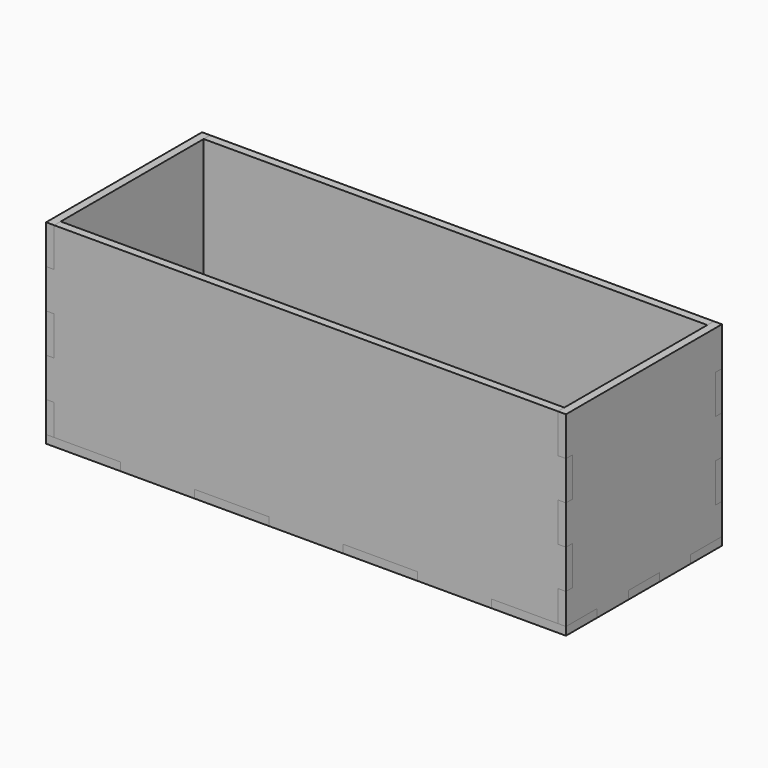
from build123d import *

# Parameters (mm, degrees)
F0_W     = 3.175
F0_H     = 3.175
F0_H_2   = 12.065
F0_W_2   = 25.8535714286
F0_H_3   = 15.24
F0_W_3   = 29.0285714286
F1_DEPTH = 3.175
F2_W     = 3.175
F2_H     = 15.24
F2_H_2   = 12.065
F2_H_3   = 3.175
F3_DEPTH = 3.175
F7_DEPTH = 3.175


with BuildPart() as f1:
    # F0 (on Top) → F1 (new body)
    with BuildSketch(Plane.XY):
        with Locations((-100.0125, 36.5125)):
            Rectangle(F0_W, F0_H)
        with Locations((-100.0125, 28.8925)):
            Rectangle(F0_W, F0_H_2)
        with Locations((-85.4982142857, 36.5125)):
            Rectangle(F0_W_2, F0_H)
        Polygon((98.425, 22.86), (98.425, 34.925), (72.5714285714, 34.925), (43.5428571429, 34.925), (14.5142857143, 34.925), (-14.5142857143, 34.925), (-43.5428571429, 34.925), (-72.5714285714, 34.925), (-98.425, 34.925), (-98.425, 22.86), (-98.425, 7.62), (-98.425, -7.62), (-98.425, -22.86), (-98.425, -34.925), (-72.5714285714, -34.925), (-43.5428571429, -34.925), (-14.5142857143, -34.925), (14.5142857143, -34.925), (43.5428571429, -34.925), (72.5714285714, -34.925), (98.425, -34.925), (98.425, -22.86), (98.425, -7.62), (98.425, 7.62), align=None)
        with Locations((-100.0125, 0)):
            Rectangle(F0_W, F0_H_3)
        with Locations((-100.0125, -28.8925)):
            Rectangle(F0_W, F0_H_2)
        with Locations((-100.0125, -36.5125)):
            Rectangle(F0_W, F0_H)
        with Locations((-85.4982142857, -36.5125)):
            Rectangle(F0_W_2, F0_H)
        with Locations((-29.0285714286, -36.5125)):
            Rectangle(F0_W_3, F0_H)
        with Locations((29.0285714286, -36.5125)):
            Rectangle(F0_W_3, F0_H)
        with Locations((85.4982142857, -36.5125)):
            Rectangle(F0_W_2, F0_H)
        with Locations((100.0125, -36.5125)):
            Rectangle(F0_W, F0_H)
        with Locations((100.0125, -28.8925)):
            Rectangle(F0_W, F0_H_2)
        with Locations((100.0125, 0)):
            Rectangle(F0_W, F0_H_3)
        with Locations((100.0125, 28.8925)):
            Rectangle(F0_W, F0_H_2)
        with Locations((100.0125, 36.5125)):
            Rectangle(F0_W, F0_H)
        with Locations((85.4982142857, 36.5125)):
            Rectangle(F0_W_2, F0_H)
        with Locations((29.0285714286, 36.5125)):
            Rectangle(F0_W_3, F0_H)
        with Locations((-29.0285714286, 36.5125)):
            Rectangle(F0_W_3, F0_H)
    extrude(amount=F1_DEPTH)


with BuildPart() as f3:
    # F2 (on face) → F3 (new body)
    with BuildSketch(Plane.YZ.offset(101.6)):
        Polygon((-22.86, 3.175), (-22.86, 0), (34.925, 0), (34.925, 15.24), (34.925, 30.48), (34.925, 45.72), (34.925, 60.96), (34.925, 76.2), (-34.925, 76.2), (-34.925, 60.96), (-34.925, 45.72), (-34.925, 30.48), (-34.925, 15.24), (-34.925, 3.175), align=None)
        with Locations((-36.5125, 68.58)):
            Rectangle(F2_W, F2_H)
        with Locations((-36.5125, 38.1)):
            Rectangle(F2_W, F2_H)
        with Locations((-36.5125, 9.2075)):
            Rectangle(F2_W, F2_H_2)
        with Locations((-36.5125, 1.5875)):
            Rectangle(F2_W, F2_H_3)
        with Locations((36.5125, 7.62)):
            Rectangle(F2_W, F2_H)
        with Locations((36.5125, 38.1)):
            Rectangle(F2_W, F2_H)
        with Locations((36.5125, 68.58)):
            Rectangle(F2_W, F2_H)
    extrude(amount=-F3_DEPTH)


with BuildPart() as f4_1:
    # F4: instance of F3
    add(f3.part.mirror(Plane.YZ))

    # F5: cut F1
    add(f1.part, mode=Mode.SUBTRACT)


with BuildPart() as f3_1:
    add(f3.part)

    # F5: cut F1
    add(f1.part, mode=Mode.SUBTRACT)


with BuildPart() as f7:
    # F6 (on face) → F7 (new body)
    with BuildSketch(Plane(origin=(0, 38.1, 0), x_dir=(-1, 0, 0), z_dir=(0, 1, 0))):
        Polygon((-72.5714285714, 3.175), (-72.5714285714, 0), (101.6, 0), (101.6, 76.2), (-101.6, 76.2), (-101.6, 3.175), align=None)
    extrude(amount=-F7_DEPTH)


with BuildPart() as f8_1:
    # F8: instance of F7
    add(f7.part.mirror(Plane.XZ))

    # F9: cut F4_1, F1, F3
    add(f4_1.part, mode=Mode.SUBTRACT)
    add(f1.part, mode=Mode.SUBTRACT)
    add(f3_1.part, mode=Mode.SUBTRACT)


with BuildPart() as f7_1:
    add(f7.part)

    # F9: cut F4_1, F1, F3
    add(f4_1.part, mode=Mode.SUBTRACT)
    add(f1.part, mode=Mode.SUBTRACT)
    add(f3_1.part, mode=Mode.SUBTRACT)


solid = Compound([f1.part, f4_1.part, f3_1.part, f8_1.part, f7_1.part])
